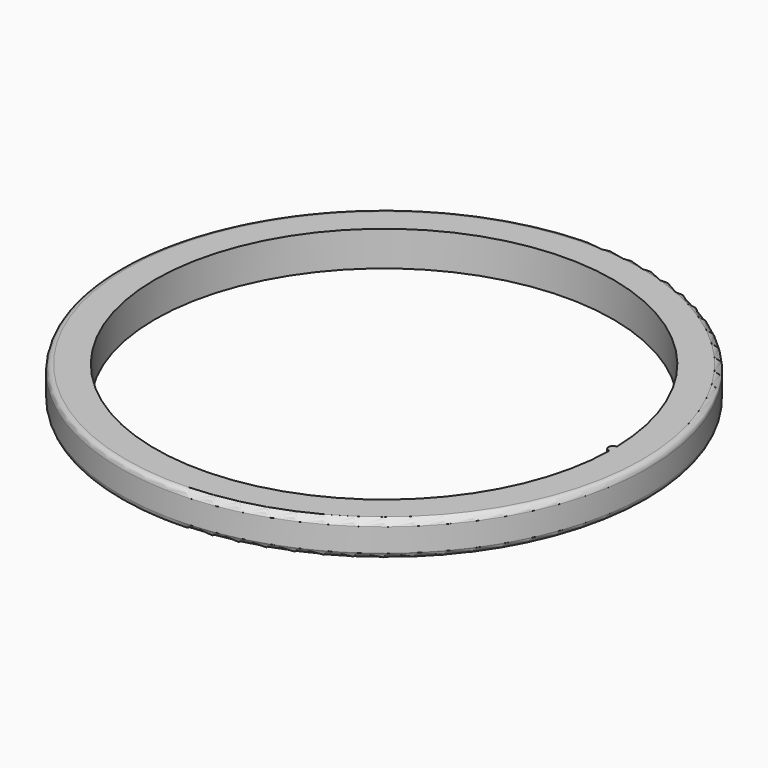
from build123d import *

# Parameters (mm, degrees)
F1_R     = 45.35
F2_DEPTH = 3
F4_R     = 1


with BuildPart() as f2:
    # F1 (on Top) → F2 (new body, symmetric)
    with BuildSketch(Plane.XY):
        Circle(F1_R)
        with BuildLine():
            ThreePointArc((39.3418678526, 0.7999586665), (39.3479669106, 0.4), (39.35, 0))
            ThreePointArc((39.35, 0), (39.3479669106, -0.4), (39.3418678526, -0.7999586665))
            ThreePointArc((39.3418678526, -0.7999586665), (-39.35, 0), (39.3418678526, 0.7999586665))
        make_face(mode=Mode.SUBTRACT)
        with BuildLine():
            ThreePointArc((39.3418678526, -0.7999586665), (39.3479669106, -0.4), (39.35, 0))
            ThreePointArc((39.35, 0), (39.3479669106, 0.4), (39.3418678526, 0.7999586665))
            ThreePointArc((39.3418678526, 0.7999586665), (38.55, 0), (39.3418678526, -0.7999586665))
        make_face()
    extrude(amount=F2_DEPTH, both=True)

    # F4
    f4_edges = [f2.edges().sort_by_distance(p)[0] for p in [
        (-45.35, 0, 3),
        (-45.35, 0, -3),
    ]]
    fillet(f4_edges, radius=F4_R)


solid = f2.part
